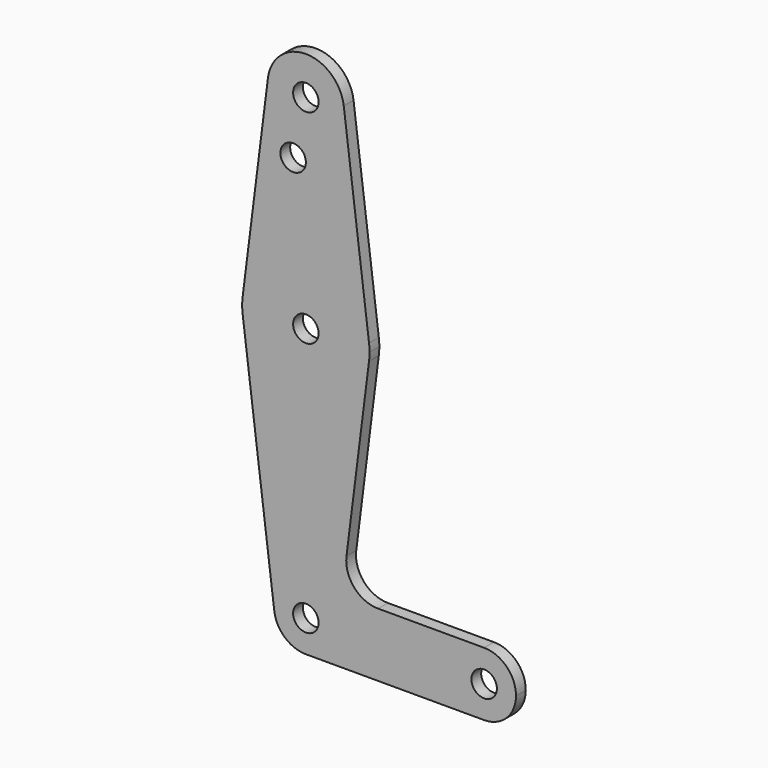
from build123d import *

# Parameters (mm, degrees)
F0_R     = 3.175
F1_DEPTH = 3.048


# Not quite as in the source:
# - a feature names something its author has since deleted; it is built from what else it names


with BuildPart() as f1:
    # F0 (on Front) → F1 (new body)
    with BuildSketch(Plane.XZ):
        with BuildLine():
            ThreePointArc((0, -7.9375), (5.6126600757, -5.6126600757), (7.9375, 0))
            ThreePointArc((7.9375, 0), (-0.4970693683, 7.9219207452), (-7.8752441368, -0.9921875))
            ThreePointArc((-7.8752441368, -0.9921875), (-5.2501627579, -5.953125), (0, -7.9375))
        make_face()
        Circle(F0_R, mode=Mode.SUBTRACT)
        with BuildLine():
            ThreePointArc((-7.8752441368, -0.9921875), (-0.4970693683, 7.9219207452), (7.9375, 0))
            ThreePointArc((7.9375, 0), (5.6126600757, -5.6126600757), (0, -7.9375))
            Line((0, -7.9375), (44.45, -7.9375))
            ThreePointArc((44.45, -7.9375), (36.5125, 0), (44.45, 7.9375))
            Line((44.45, 7.9375), (18.0149584735, 7.9375))
            ThreePointArc((18.0149584735, 7.9375), (12.0523084735, 10.6291369817), (10.127113946, 16.881475))
            Line((10.127113946, 16.881475), (15.7504882737, 61.515625))
            ThreePointArc((15.7504882737, 61.515625), (0, 47.625), (-15.7504882737, 61.515625))
            Line((-15.7504882737, 61.515625), (-7.8752441368, -0.9921875))
        make_face()
        with BuildLine():
            ThreePointArc((-15.7504882737, 65.484375), (-15.875, 63.5), (-15.7504882737, 61.515625))
            ThreePointArc((-15.7504882737, 61.515625), (0, 47.625), (15.7504882737, 61.515625))
            ThreePointArc((15.7504882737, 61.515625), (15.8438414904, 62.5058612634), (15.875, 63.5))
            ThreePointArc((15.875, 63.5), (15.8438414904, 64.4941387366), (15.7504882737, 65.484375))
            ThreePointArc((15.7504882737, 65.484375), (0, 79.375), (-15.7504882737, 65.484375))
        make_face()
        with Locations((0, 63.5)):
            Circle(F0_R, mode=Mode.SUBTRACT)
        with BuildLine():
            ThreePointArc((44.45, 7.9375), (36.5125, 0), (44.45, -7.9375))
            ThreePointArc((44.45, -7.9375), (50.0626600757, -5.6126600757), (52.3875, 0))
            ThreePointArc((52.3875, 0), (50.0626600757, 5.6126600757), (44.45, 7.9375))
        make_face()
        with Locations((44.45, 0)):
            Circle(F0_R, mode=Mode.SUBTRACT)
        with BuildLine():
            Line((-9.4502929642, 115.490625), (-15.7504882737, 65.484375))
            ThreePointArc((-15.7504882737, 65.484375), (0, 79.375), (15.7504882737, 65.484375))
            Line((15.7504882737, 65.484375), (9.4502929642, 115.490625))
            ThreePointArc((9.4502929642, 115.490625), (9.5063048942, 114.896483242), (9.525, 114.3))
            ThreePointArc((9.525, 114.3), (-0.596483242, 104.7936951058), (-9.4502929642, 115.490625))
        make_face()
        with Locations((-3.175, 100.0252)):
            Circle(F0_R, mode=Mode.SUBTRACT)
        with BuildLine():
            ThreePointArc((9.4502929642, 115.490625), (0, 123.825), (-9.4502929642, 115.490625))
            ThreePointArc((-9.4502929642, 115.490625), (-0.596483242, 104.7936951058), (9.525, 114.3))
            ThreePointArc((9.525, 114.3), (9.5063048942, 114.896483242), (9.4502929642, 115.490625))
        make_face()
        with Locations((0, 114.3)):
            Circle(F0_R, mode=Mode.SUBTRACT)
    extrude(amount=F1_DEPTH)


solid = f1.part
